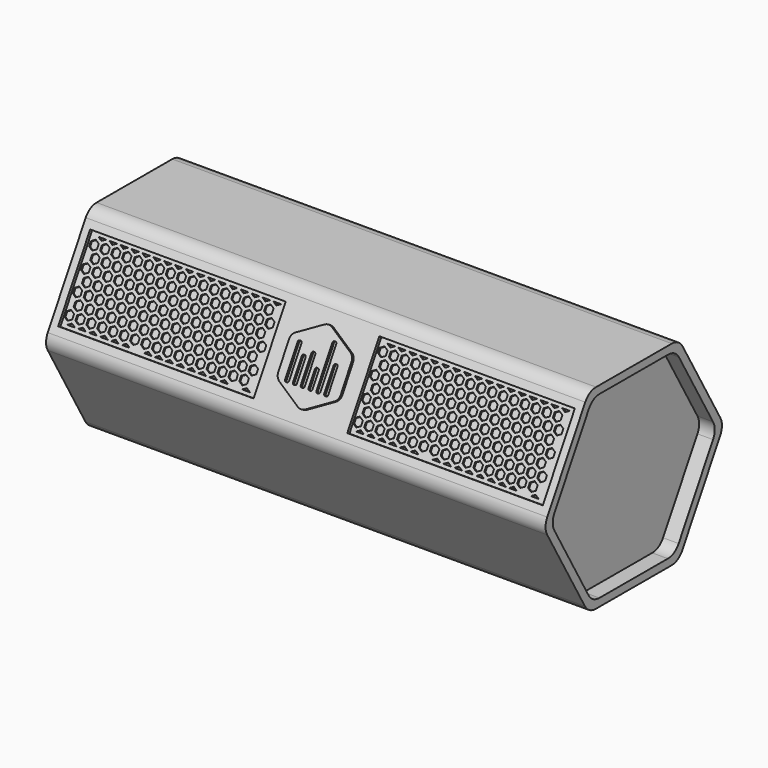
from build123d import *

# Parameters (mm, degrees)
F1_DEPTH  = 320
F3_DEPTH  = 1.5
F4_R      = 10
F6_DEPTH  = 10
F8_DEPTH  = 10
F9_R      = 10
F10_R     = 5
F11_W     = 125.25
F11_H     = 51.1217782649
F12_DEPTH = 3
F13_DEPTH = 3
F14_DEPTH = 1
F16_DEPTH = 1
F18_W     = 2.5
F18_H     = 22
F18_H_2   = 16
F18_H_3   = 19
F18_H_4   = 12
F18_H_5   = 27.5
F18_H_6   = 17
F19_DEPTH = 2
F20_R     = 1


with BuildPart() as f1:
    # F0 (on Right) → F1 (new body)
    with BuildSketch(Plane.YZ):
        Polygon((-35.9565990903, 62.5736071774), (-72.1686329672, 0.1474753428), (-36.2120338769, -62.4261318346), (35.9565990903, -62.5736071774), (72.1686329672, -0.1474753428), (36.2120338769, 62.4261318346), align=None)
    extrude(amount=F1_DEPTH)

    # F4
    f4_edges = [f1.edges().sort_by_distance(p)[0] for p in [
        (160, 36.212034, 62.426132),
        (160, -35.956599, 62.573607),
        (160, -72.168633, 0.147475),
        (160, -36.212034, -62.426132),
        (160, 35.956599, -62.573607),
        (160, 72.168633, -0.147475),
    ]]
    fillet(f4_edges, radius=F4_R)

    # F5 (on face) → F6 (cut)
    with BuildSketch(Plane(origin=(0, 0, 0), x_dir=(0, -1, 0), z_dir=(-1, 0, 0))):
        Polygon((33.207939238, 57.4942419201), (-33.1875044551, 57.5060399475), (-66.3954436931, 0.0117980274), (-33.207939238, -57.4942419201), (33.1875044551, -57.5060399475), (66.3954436931, -0.0117980274), align=None)
    extrude(amount=-F6_DEPTH, mode=Mode.SUBTRACT)

    # F7 (on face) → F8 (cut)
    with BuildSketch(Plane.YZ.offset(320)):
        Polygon((33.3252825309, 57.4261318346), (-33.0698477444, 57.5736071774), (-66.3951302753, 0.1474753428), (-33.3252825309, -57.4261318346), (33.0698477444, -57.5736071774), (66.3951302753, -0.1474753428), align=None)
    extrude(amount=-F8_DEPTH, mode=Mode.SUBTRACT)

    # F9
    f9_edges = [f1.edges().sort_by_distance(p)[0] for p in [
        (5, 33.187504, 57.50604),
        (5, 66.395444, 0.011798),
        (5, -33.207939, 57.494242),
        (5, -66.395444, -0.011798),
        (5, -33.187504, -57.50604),
        (5, 33.207939, -57.494242),
        (315, 33.325283, 57.426132),
        (315, 66.39513, -0.147475),
        (315, -33.069848, 57.573607),
        (315, -66.39513, 0.147475),
        (315, -33.325283, -57.426132),
        (315, 33.069848, -57.573607),
    ]]
    fillet(f9_edges, radius=F9_R)

    # F11 (on face) → F12 (cut)
    with BuildSketch(Plane(origin=(0, -54.0626160288, 31.3605412601), x_dir=(1, 0, 0), z_dir=(0, -0.8650018565, 0.5017686602))):
        with Locations((67.375, 0)):
            Rectangle(F11_W, F11_H)
    extrude(amount=-F12_DEPTH, mode=Mode.SUBTRACT)

    # F11 (on face) → F13 (cut)
    with BuildSketch(Plane(origin=(0, -54.0626160288, 31.3605412601), x_dir=(1, 0, 0), z_dir=(0, -0.8650018565, 0.5017686602))):
        with Locations((252.625, 0)):
            Rectangle(F11_W, F11_H)
    extrude(amount=-F13_DEPTH, mode=Mode.SUBTRACT)


with BuildPart() as f3:
    # F2 (on face) → F3 (new body)
    with BuildSketch(Plane(origin=(0, -54.0626160288, 31.3605412601), x_dir=(1, 0, 0), z_dir=(0, -0.8650018565, 0.5017686602))):
        Polygon((159.8552660133, 23.0669244835), (139.9510904167, 11.4081189325), (140.0958244034, -11.658805551), (160.1447339867, -23.0669244835), (180.0489095833, -11.4081189325), (179.9041755966, 11.658805551), align=None)
    extrude(amount=F3_DEPTH)

    # F10
    f10_edges = [f3.edges().sort_by_distance(p)[0] for p in [
        (159.855266, -43.137108, 51.6898),
        (179.904176, -48.861344, 41.821756),
        (180.04891, -60.435604, 21.868824),
        (160.144734, -66.285627, 11.783935),
        (140.095824, -60.561391, 21.651979),
        (139.95109, -48.987131, 41.604912),
    ]]
    fillet(f10_edges, radius=F10_R)

    # F18 (on face) → F19 (cut)
    with BuildSketch(Plane(origin=(0, -55.3601188135, 32.1131942503), x_dir=(1, 0, 0), z_dir=(0, -0.8650018565, 0.5017686602))):
        with Locations((146.6441166401, -1.09411787)):
            Rectangle(F18_W, F18_H)
        with Locations((151.6441166401, -4.0627452467)):
            Rectangle(F18_W, F18_H_2)
        with Locations((156.6441166401, -2.5313726233)):
            Rectangle(F18_W, F18_H_3)
        with Locations((161.6441166401, -6)):
            Rectangle(F18_W, F18_H_4)
        with Locations((166.6441166401, 1.7813726233)):
            Rectangle(F18_W, F18_H_5)
        with Locations((171.6441166401, -3.4372547533)):
            Rectangle(F18_W, F18_H_6)
    extrude(amount=-F19_DEPTH, mode=Mode.SUBTRACT)

    # F20
    f20_edges = [f3.edges().sort_by_distance(p)[0] for p in [
        (145.394117, -49.740906, 40.305474),
        (147.894117, -49.740906, 40.305474),
        (145.394117, -60.779817, 21.275433),
        (147.894117, -60.779817, 21.275433),
        (150.394117, -52.735776, 35.1426),
        (152.894117, -52.735776, 35.1426),
        (152.894117, -60.764075, 21.302571),
        (150.394117, -60.764075, 21.302571),
        (155.394117, -51.214729, 37.764743),
        (157.894117, -51.214729, 37.764743),
        (157.894117, -60.748333, 21.329708),
        (155.394117, -60.748333, 21.329708),
        (160.394117, -54.711367, 31.736868),
        (162.894117, -54.711367, 31.736868),
        (162.894117, -60.732591, 21.356845),
        (160.394117, -60.732591, 21.356845),
        (165.394117, -46.918211, 45.171534),
        (167.894117, -46.918211, 45.171534),
        (167.894117, -60.71685, 21.383983),
        (165.394117, -60.71685, 21.383983),
        (172.894117, -52.171041, 36.116152),
        (170.394117, -52.171041, 36.116152),
        (172.894117, -60.701108, 21.41112),
        (170.394117, -60.701108, 21.41112),
    ]]
    fillet(f20_edges, radius=F20_R)


with BuildPart() as f14:
    # F14 (new): a face of the model
    f14_faces = [f1.part.faces().sort_by_distance(p)[0] for p in [
        (67.375, -51.4676104594, 29.8552352796),
    ]]
    extrude(f14_faces, amount=F14_DEPTH)

    # F15 (on face) → F16 (cut)
    with BuildSketch(Plane(origin=(0, -52.3326123159, 30.3570039398), x_dir=(1, 0, 0), z_dir=(0, -0.8650018565, 0.5017686602))):
        Polygon((69.875, -1.443375673), (69.875, 1.443375673), (67.375, 2.8867513459), (64.875, 1.443375673), (64.875, -1.443375673), (67.375, -2.8867513459), align=None)
        Polygon((74.3182979262, 2.8861944162), (71.8471312784, 1.3939917717), (71.9038333522, -1.4922026445), (74.4317020738, -2.8861944162), (76.9028687216, -1.3939917717), (76.8461666478, 1.4922026445), align=None)
        Polygon((81.375, 2.8867513459), (78.875, 1.443375673), (78.875, -1.443375673), (81.375, -2.8867513459), (83.875, -1.443375673), (83.875, 1.443375673), align=None)
        Polygon((88.375, 2.886751346), (85.875, 1.443375673), (85.875, -1.443375673), (88.375, -2.8867513459), (90.875, -1.443375673), (90.875, 1.443375673), align=None)
        Polygon((95.375, 2.8867513459), (92.875, 1.443375673), (92.875, -1.443375673), (95.375, -2.8867513459), (97.875, -1.443375673), (97.875, 1.443375673), align=None)
        Polygon((102.375, 2.8867513459), (99.875, 1.443375673), (99.875, -1.443375673), (102.375, -2.886751346), (104.875, -1.443375673), (104.875, 1.443375673), align=None)
        Polygon((109.375, 2.8867513459), (106.875, 1.443375673), (106.875, -1.443375673), (109.375, -2.8867513459), (111.875, -1.443375673), (111.875, 1.443375673), align=None)
        Polygon((116.375, 2.8867513459), (113.875, 1.443375673), (113.875, -1.443375673), (116.375, -2.8867513459), (118.875, -1.443375673), (118.875, 1.443375673), align=None)
        Polygon((123.375, 2.8867513459), (120.875, 1.4433756729), (120.875, -1.443375673), (123.375, -2.886751346), (125.875, -1.443375673), (125.875, 1.4433756729), align=None)
        Polygon((22.875, -1.443375673), (25.375, -2.8867513459), (27.875, -1.443375673), (27.875, 1.443375673), (25.375, 2.8867513459), (22.875, 1.443375673), align=None)
        Polygon((20.875, -1.443375673), (20.875, 1.443375673), (18.375, 2.8867513459), (15.875, 1.443375673), (15.875, -1.443375673), (18.375, -2.8867513459), align=None)
        Polygon((29.875, -1.443375673), (32.375, -2.886751346), (34.875, -1.443375673), (34.875, 1.443375673), (32.375, 2.8867513459), (29.875, 1.443375673), align=None)
        Polygon((13.875, 1.4433756729), (11.375, 2.8867513459), (8.875, 1.4433756729), (8.875, -1.443375673), (11.375, -2.886751346), (13.875, -1.443375673), align=None)
        Polygon((48.875, 1.443375673), (46.375, 2.886751346), (43.875, 1.443375673), (43.875, -1.443375673), (46.375, -2.8867513459), (48.875, -1.443375673), align=None)
        Polygon((50.875, -1.443375673), (53.375, -2.8867513459), (55.875, -1.443375673), (55.875, 1.443375673), (53.375, 2.8867513459), (50.875, 1.443375673), align=None)
        Polygon((41.875, -1.443375673), (41.875, 1.443375673), (39.375, 2.8867513459), (36.875, 1.443375673), (36.875, -1.443375673), (39.375, -2.8867513459), align=None)
        Polygon((62.9028687216, 1.3939917717), (60.4317020738, 2.8861944162), (57.9038333522, 1.4922026445), (57.8471312784, -1.3939917717), (60.3182979262, -2.8861944162), (62.8461666478, -1.4922026445), align=None)
        Polygon((50.2418052453, 9.1463911622), (47.7418052453, 7.7030154892), (47.7418052453, 4.8162641432), (50.2418052453, 3.3728884703), (52.7418052453, 4.8162641432), (52.7418052453, 7.7030154892), align=None)
        Polygon((106.2418052453, 9.1463911622), (103.7418052453, 7.7030154892), (103.7418052453, 4.8162641432), (106.2418052453, 3.3728884703), (108.7418052453, 4.8162641432), (108.7418052453, 7.7030154892), align=None)
        Polygon((8.2418052453, 9.1463911621), (8.2418052453, 3.3728884702), (10.7418052453, 4.8162641432), (10.7418052453, 7.7030154892), align=None)
        Polygon((5.7418052453, 4.8162641432), (8.2418052453, 3.3728884702), (8.2418052453, 9.1463911621), (5.7418052453, 7.7030154891), align=None)
        Polygon((117.7418052453, 4.8162641432), (120.2418052452, 3.3728884702), (122.7418052452, 4.8162641432), (122.7418052453, 7.7030154891), (120.2418052453, 9.1463911621), (117.7418052453, 7.7030154892), align=None)
        Polygon((22.2418052453, 9.1463911622), (19.7418052453, 7.7030154892), (19.7418052453, 4.8162641432), (22.2418052453, 3.3728884703), (24.7418052453, 4.8162641432), (24.7418052453, 7.7030154892), align=None)
        Polygon((38.7418052453, 4.8162641433), (38.7418052453, 7.7030154892), (36.2418052453, 9.1463911622), (33.7418052453, 7.7030154892), (33.7418052453, 4.8162641432), (36.2418052453, 3.3728884703), align=None)
        Polygon((92.2418052453, 9.1463911622), (89.7418052453, 7.7030154892), (89.7418052453, 4.8162641433), (92.2418052453, 3.3728884703), (94.7418052453, 4.8162641432), (94.7418052453, 7.7030154892), align=None)
        Polygon((99.2418052453, 9.1463911622), (96.7418052453, 7.7030154892), (96.7418052453, 4.8162641432), (99.2418052453, 3.3728884703), (101.7418052453, 4.8162641432), (101.7418052453, 7.7030154892), align=None)
        Polygon((64.2418052453, 3.3728884703), (66.7418052453, 4.8162641433), (66.7418052453, 7.7030154892), (64.2418052453, 9.1463911622), (61.7418052453, 7.7030154892), (61.7418052453, 4.8162641432), align=None)
        Polygon((115.7418052453, 4.8162641432), (115.7418052453, 7.7030154892), (113.2418052453, 9.1463911622), (110.7418052453, 7.7030154892), (110.7418052453, 4.8162641432), (113.2418052453, 3.3728884703), align=None)
        Polygon((43.2418052453, 9.1463911622), (40.7418052453, 7.7030154892), (40.7418052453, 4.8162641433), (43.2418052453, 3.3728884703), (45.7418052453, 4.8162641433), (45.7418052453, 7.7030154892), align=None)
        Polygon((82.7418052453, 4.8162641433), (85.2418052453, 3.3728884703), (87.7418052453, 4.8162641433), (87.7418052453, 7.7030154892), (85.2418052453, 9.1463911622), (82.7418052453, 7.7030154892), align=None)
        Polygon((75.7418052453, 4.8162641432), (78.2418052453, 3.3728884703), (80.7418052453, 4.8162641432), (80.7418052453, 7.7030154892), (78.2418052453, 9.1463911622), (75.7418052453, 7.7030154892), align=None)
        Polygon((59.712971893, 4.7674371717), (59.7696739669, 7.6536315879), (57.2985073191, 9.1458342324), (54.7706385975, 7.7518424607), (54.7139365236, 4.8656480445), (57.1851031714, 3.3734454), align=None)
        Polygon((26.7418052453, 4.8162641432), (29.2418052453, 3.3728884703), (31.7418052453, 4.8162641432), (31.7418052453, 7.7030154892), (29.2418052453, 9.1463911622), (26.7418052453, 7.7030154892), align=None)
        Polygon((17.7418052453, 7.7030154892), (15.2418052453, 9.1463911622), (12.7418052453, 7.7030154892), (12.7418052453, 4.8162641432), (15.2418052453, 3.3728884703), (17.7418052453, 4.8162641432), align=None)
        Polygon((71.2985073191, 3.3734454), (73.7696739669, 4.8656480445), (73.712971893, 7.7518424607), (71.1851031714, 9.1458342324), (68.7139365236, 7.6536315879), (68.7706385975, 4.7674371717), align=None)
        Polygon((123.7049438918, 9.5428702504), (126.2049438918, 10.9862459233), (126.2049438918, 13.8729972693), (123.7049438918, 15.3163729422), (121.2049438918, 13.8729972693), (121.2049438918, 10.9862459233), align=None)
        Polygon((32.7049438918, 15.3163729423), (30.2049438918, 13.8729972693), (30.2049438918, 10.9862459234), (32.7049438918, 9.5428702504), (35.2049438918, 10.9862459234), (35.2049438918, 13.8729972693), align=None)
        Polygon((116.7049438918, 9.5428702504), (119.2049438918, 10.9862459234), (119.2049438918, 13.8729972693), (116.7049438918, 15.3163729423), (114.2049438918, 13.8729972693), (114.2049438918, 10.9862459234), align=None)
        Polygon((27.0717491371, 17.2458857396), (29.5717491371, 15.8025100666), (32.0717491371, 17.2458857396), (32.0717491371, 20.1326370855), (29.5717491371, 21.5760127585), (27.0717491371, 20.1326370855), align=None)
        Polygon((56.2049438918, 10.9862459234), (56.2049438918, 13.8729972693), (53.7049438918, 15.3163729423), (51.2049438918, 13.8729972693), (51.2049438918, 10.9862459234), (53.7049438918, 9.5428702504), align=None)
        Polygon((18.7049438918, 9.5428702504), (21.2049438918, 10.9862459234), (21.2049438918, 13.8729972693), (18.7049438918, 15.3163729423), (16.2049438918, 13.8729972693), (16.2049438918, 10.9862459234), align=None)
        Polygon((88.7049438918, 9.5428702504), (91.2049438918, 10.9862459234), (91.2049438918, 13.8729972693), (88.7049438918, 15.3163729423), (86.2049438918, 13.8729972693), (86.2049438918, 10.9862459234), align=None)
        Polygon((22.5717491371, 21.5760127585), (20.0717491371, 20.1326370855), (20.0717491371, 17.2458857396), (22.5717491371, 15.8025100666), (25.0717491371, 17.2458857396), (25.0717491371, 20.1326370855), align=None)
        Polygon((120.5717491371, 15.8025100666), (123.0717491371, 17.2458857395), (123.0717491371, 20.1326370855), (120.5717491371, 21.5760127585), (118.0717491371, 20.1326370855), (118.0717491371, 17.2458857396), align=None)
        Polygon((23.2049438918, 10.9862459234), (25.7049438918, 9.5428702504), (28.2049438918, 10.9862459234), (28.2049438918, 13.8729972693), (25.7049438918, 15.3163729423), (23.2049438918, 13.8729972693), align=None)
        Polygon((37.2049438918, 13.8729972693), (37.2049438918, 10.9862459234), (39.7049438918, 9.5428702504), (42.2049438918, 10.9862459234), (42.2049438918, 13.8729972693), (39.7049438918, 15.3163729423), align=None)
        Polygon((49.2049438918, 10.9862459234), (49.2049438918, 13.8729972693), (46.7049438918, 15.3163729423), (44.2049438918, 13.8729972693), (44.2049438918, 10.9862459234), (46.7049438918, 9.5428702504), align=None)
        Polygon((11.7049438918, 15.3163729422), (9.2049438918, 13.8729972693), (9.2049438919, 10.9862459233), (11.7049438919, 9.5428702504), (14.2049438918, 10.9862459233), (14.2049438918, 13.8729972693), align=None)
        Polygon((83.0717491371, 17.2458857396), (85.5717491371, 15.8025100666), (88.0717491371, 17.2458857396), (88.0717491371, 20.1326370855), (85.5717491371, 21.5760127585), (83.0717491371, 20.1326370855), align=None)
        Polygon((81.7049438918, 15.3163729423), (79.2049438918, 13.8729972693), (79.2049438918, 10.9862459234), (81.7049438918, 9.5428702504), (84.2049438918, 10.9862459234), (84.2049438918, 13.8729972693), align=None)
        Polygon((60.7616459657, 15.3158160125), (58.2337772441, 13.9218242408), (58.1770751702, 11.0356298246), (60.648241818, 9.5434271801), (63.1761105396, 10.9374189518), (63.2328126135, 13.8236133681), align=None)
        Polygon((74.0429157849, 20.1814640571), (71.5150470633, 21.5754558288), (69.0438804155, 20.0832531843), (69.1005824893, 17.1970587681), (71.6284512109, 15.8030669964), (74.0996178587, 17.2952696408), align=None)
        Polygon((50.5717491371, 15.8025100666), (53.0717491371, 17.2458857396), (53.0717491371, 20.1326370855), (50.5717491371, 21.5760127585), (48.0717491371, 20.1326370855), (48.0717491371, 17.2458857396), align=None)
        Polygon((65.2049438918, 10.9862459234), (67.7049438918, 9.5428702504), (70.2049438918, 10.9862459234), (70.2049438918, 13.8729972693), (67.7049438918, 15.3163729423), (65.2049438918, 13.8729972693), align=None)
        Polygon((109.0717491371, 17.2458857396), (109.0717491371, 20.1326370855), (106.5717491371, 21.5760127585), (104.0717491371, 20.1326370855), (104.0717491371, 17.2458857396), (106.5717491371, 15.8025100666), align=None)
        Polygon((102.7049438918, 9.5428702504), (105.2049438918, 10.9862459234), (105.2049438918, 13.8729972693), (102.7049438918, 15.3163729423), (100.2049438918, 13.8729972693), (100.2049438918, 10.9862459234), align=None)
        Polygon((43.5717491371, 21.5760127585), (41.0717491371, 20.1326370855), (41.0717491371, 17.2458857396), (43.5717491371, 15.8025100666), (46.0717491371, 17.2458857396), (46.0717491371, 20.1326370855), align=None)
        Polygon((112.2049438918, 13.8729972693), (109.7049438918, 15.3163729423), (107.2049438918, 13.8729972693), (107.2049438918, 10.9862459234), (109.7049438918, 9.5428702504), (112.2049438918, 10.9862459234), align=None)
        Polygon((67.0717491371, 20.1326370855), (64.5717491371, 21.5760127585), (62.0717491371, 20.1326370855), (62.0717491371, 17.2458857396), (64.5717491371, 15.8025100666), (67.0717491371, 17.2458857396), align=None)
        Polygon((18.0717491371, 20.1326370855), (15.5717491371, 21.5760127585), (13.0717491371, 20.1326370855), (13.0717491371, 17.2458857396), (15.5717491371, 15.8025100666), (18.0717491371, 17.2458857396), align=None)
        Polygon((98.2049438918, 13.8729972693), (95.7049438918, 15.3163729423), (93.2049438918, 13.8729972693), (93.2049438918, 10.9862459234), (95.7049438918, 9.5428702504), (98.2049438918, 10.9862459234), align=None)
        Polygon((92.5717491371, 15.8025100666), (95.0717491371, 17.2458857396), (95.0717491371, 20.1326370855), (92.5717491371, 21.5760127585), (90.0717491371, 20.1326370855), (90.0717491371, 17.2458857396), align=None)
        Polygon((72.2337772441, 10.9374189519), (74.7616459657, 9.5434271801), (77.2328126135, 11.0356298246), (77.1761105396, 13.9218242408), (74.648241818, 15.3158160125), (72.1770751702, 13.8236133681), align=None)
        Polygon((55.0438804155, 17.2952696408), (57.5150470633, 15.8030669964), (60.0429157849, 17.1970587681), (60.0996178587, 20.0832531843), (57.6284512109, 21.5754558288), (55.1005824893, 20.1814640571), align=None)
        Polygon((81.0717491371, 20.1326370855), (78.5717491371, 21.5760127585), (76.0717491371, 20.1326370855), (76.0717491371, 17.2458857396), (78.5717491371, 15.8025100666), (81.0717491371, 17.2458857396), align=None)
        Polygon((8.5717491371, 21.5760127585), (6.0717491371, 20.1326370855), (6.0717491371, 17.2458857395), (8.5717491371, 15.8025100666), align=None)
        Polygon((11.0717491371, 20.1326370855), (8.5717491371, 21.5760127585), (8.5717491371, 15.8025100666), (11.0717491371, 17.2458857396), align=None)
        Polygon((99.5717491371, 21.5760127585), (97.0717491371, 20.1326370855), (97.0717491371, 17.2458857396), (99.5717491371, 15.8025100666), (102.0717491371, 17.2458857396), (102.0717491371, 20.1326370855), align=None)
        Polygon((36.5717491371, 15.8025100666), (39.0717491371, 17.2458857396), (39.0717491371, 20.1326370855), (36.5717491371, 21.5760127585), (34.0717491371, 20.1326370855), (34.0717491371, 17.2458857396), align=None)
        Polygon((111.0717491371, 17.2458857396), (113.5717491371, 15.8025100666), (116.0717491371, 17.2458857396), (116.0717491371, 20.1326370855), (113.5717491371, 21.5760127585), (111.0717491371, 20.1326370855), align=None)
        Polygon((124.0348877837, 21.9724918467), (126.5348877837, 23.4158675197), (121.5348877837, 23.4158675197), align=None)
        Polygon((117.0348877837, 21.9724918467), (119.5348877837, 23.4158675197), (114.5348877837, 23.4158675197), align=None)
        Polygon((56.5348877837, 23.4158675197), (51.5348877837, 23.4158675197), (54.0348877837, 21.9724918467), align=None)
        Polygon((89.0348877837, 21.9724918467), (91.5348877837, 23.4158675197), (86.5348877837, 23.4158675197), align=None)
        Polygon((23.5348877837, 23.4158675197), (26.0348877837, 21.9724918467), (28.5348877837, 23.4158675197), align=None)
        Polygon((42.5348877837, 23.4158675197), (37.5348877837, 23.4158675197), (40.0348877837, 21.9724918467), align=None)
        Polygon((49.5348877837, 23.4158675197), (44.5348877837, 23.4158675197), (47.0348877837, 21.9724918467), align=None)
        Polygon((21.5348877837, 23.4158675197), (16.5348877837, 23.4158675197), (19.0348877837, 21.9724918467), align=None)
        Polygon((79.5348877837, 23.4158675197), (82.0348877837, 21.9724918467), (84.5348877837, 23.4158675197), align=None)
        Polygon((65.5348877837, 23.4158675197), (68.0348877837, 21.9724918467), (70.5348877837, 23.4158675197), align=None)
        Polygon((103.0348877837, 21.9724918467), (105.5348877837, 23.4158675197), (100.5348877837, 23.4158675197), align=None)
        Polygon((63.5060544315, 23.3670405482), (58.5070190621, 23.465251421), (60.9781857099, 21.9730487765), align=None)
        Polygon((110.0348877837, 21.9724918467), (112.5348877837, 23.4158675197), (107.5348877837, 23.4158675197), align=None)
        Polygon((93.5348877837, 23.4158675197), (96.0348877837, 21.9724918467), (98.5348877837, 23.4158675197), align=None)
        Polygon((72.5637211359, 23.3670405482), (75.0915898575, 21.9730487765), (77.5627565053, 23.465251421), align=None)
        Polygon((9.5348877837, 23.4158675197), (12.0348877837, 21.9724918467), (14.5348877837, 23.4158675197), align=None)
        Polygon((30.5348877837, 23.4158675197), (33.0348877837, 21.9724918467), (35.5348877837, 23.4158675197), align=None)
        Polygon((24.4695560985, -7.6147549784), (24.4695560985, -4.7280036324), (21.9695560985, -3.2846279594), (19.4695560985, -4.7280036324), (19.4695560985, -7.6147549784), (21.9695560985, -9.0581306513), align=None)
        Polygon((77.9695560985, -3.2846279594), (75.4695560985, -4.7280036324), (75.4695560985, -7.6147549784), (77.9695560985, -9.0581306513), (80.4695560985, -7.6147549784), (80.4695560985, -4.7280036324), align=None)
        Polygon((54.4983894507, -4.6791766609), (54.4416873769, -7.5653710771), (56.9128540247, -9.0575737216), (59.4407227463, -7.6635819499), (59.4974248201, -4.7773875337), (57.0262581724, -3.2851848892), align=None)
        Polygon((46.1027508533, -15.3177704676), (48.6027508533, -13.8743947946), (48.6027508533, -10.9876434486), (46.1027508533, -9.5442677757), (43.6027508533, -10.9876434486), (43.6027508533, -13.8743947946), align=None)
        Polygon((20.6027508533, -13.8743947946), (20.6027508533, -10.9876434486), (18.1027508533, -9.5442677757), (15.6027508533, -10.9876434486), (15.6027508533, -13.8743947946), (18.1027508533, -15.3177704676), align=None)
        Polygon((50.6027508533, -13.8743947946), (53.1027508533, -15.3177704676), (55.6027508533, -13.8743947946), (55.6027508533, -10.9876434486), (53.1027508533, -9.5442677757), (50.6027508533, -10.9876434486), align=None)
        Polygon((110.4695560985, -4.7280036324), (110.4695560985, -7.6147549784), (112.9695560985, -9.0581306513), (115.4695560985, -7.6147549784), (115.4695560985, -4.7280036324), (112.9695560985, -3.2846279594), align=None)
        Polygon((61.4695560985, -4.7280036324), (61.4695560985, -7.6147549784), (63.9695560985, -9.0581306513), (66.4695560985, -7.6147549784), (66.4695560985, -4.7280036324), (63.9695560985, -3.2846279594), align=None)
        Polygon((94.4695560985, -7.6147549784), (94.4695560985, -4.7280036324), (91.9695560985, -3.2846279594), (89.4695560985, -4.7280036324), (89.4695560985, -7.6147549784), (91.9695560985, -9.0581306513), align=None)
        Polygon((7.9695560985, -3.2846279595), (5.4695560985, -4.7280036325), (5.4695560985, -7.6147549784), (7.9695560985, -9.0581306514), align=None)
        Polygon((10.4695560985, -4.7280036325), (7.9695560985, -3.2846279595), (7.9695560985, -9.0581306514), (10.4695560985, -7.6147549784), align=None)
        Polygon((40.4695560985, -4.7280036324), (40.4695560985, -7.6147549784), (42.9695560985, -9.0581306513), (45.4695560985, -7.6147549784), (45.4695560985, -4.7280036324), (42.9695560985, -3.2846279594), align=None)
        Polygon((105.9695560985, -3.2846279595), (103.4695560985, -4.7280036324), (103.4695560985, -7.6147549784), (105.9695560985, -9.0581306513), (108.4695560985, -7.6147549784), (108.4695560985, -4.7280036324), align=None)
        Polygon((74.1594529271, -15.3172135378), (76.6306195749, -13.8250108933), (76.573917501, -10.9388164771), (74.0460487794, -9.5448247054), (71.5748821316, -11.0370273499), (71.6315842055, -13.9232217661), align=None)
        Polygon((99.6027508533, -13.8743947946), (102.1027508533, -15.3177704676), (104.6027508533, -13.8743947946), (104.6027508533, -10.9876434486), (102.1027508533, -9.5442677757), (99.6027508533, -10.9876434487), align=None)
        Polygon((73.4974248201, -7.5653710771), (73.4407227463, -4.6791766609), (70.9128540247, -3.2851848892), (68.4416873769, -4.7773875337), (68.4983894507, -7.6635819499), (71.0262581724, -9.0575737216), align=None)
        Polygon((39.1027508533, -9.5442677757), (36.6027508533, -10.9876434486), (36.6027508533, -13.8743947946), (39.1027508533, -15.3177704676), (41.6027508533, -13.8743947946), (41.6027508533, -10.9876434486), align=None)
        Polygon((67.1027508533, -9.5442677757), (64.6027508533, -10.9876434486), (64.6027508533, -13.8743947946), (67.1027508533, -15.3177704676), (69.6027508533, -13.8743947946), (69.6027508533, -10.9876434486), align=None)
        Polygon((32.1027508533, -15.3177704676), (34.6027508533, -13.8743947946), (34.6027508533, -10.9876434487), (32.1027508533, -9.5442677757), (29.6027508533, -10.9876434486), (29.6027508533, -13.8743947946), align=None)
        Polygon((57.5748821317, -13.8250108933), (60.0460487794, -15.3172135378), (62.573917501, -13.9232217661), (62.6306195749, -11.0370273499), (60.1594529271, -9.5448247054), (57.6315842055, -10.9388164771), align=None)
        Polygon((13.6027508533, -10.9876434487), (11.1027508533, -9.5442677757), (8.6027508533, -10.9876434487), (8.6027508533, -13.8743947946), (11.1027508533, -15.3177704676), (13.6027508533, -13.8743947946), align=None)
        Polygon((52.4695560985, -4.7280036324), (49.9695560985, -3.2846279594), (47.4695560985, -4.7280036324), (47.4695560985, -7.6147549784), (49.9695560985, -9.0581306513), (52.4695560985, -7.6147549784), align=None)
        Polygon((122.4695560985, -4.7280036325), (119.9695560985, -3.2846279595), (117.4695560985, -4.7280036325), (117.4695560985, -7.6147549784), (119.9695560985, -9.0581306514), (122.4695560985, -7.6147549784), align=None)
        Polygon((27.6027508533, -13.8743947946), (27.6027508533, -10.9876434486), (25.1027508533, -9.5442677757), (22.6027508533, -10.9876434486), (22.6027508533, -13.8743947946), (25.1027508533, -15.3177704676), align=None)
        Polygon((28.9695560985, -3.2846279595), (26.4695560985, -4.7280036324), (26.4695560985, -7.6147549784), (28.9695560985, -9.0581306513), (31.4695560985, -7.6147549784), (31.4695560985, -4.7280036324), align=None)
        Polygon((35.9695560985, -9.0581306513), (38.4695560985, -7.6147549784), (38.4695560985, -4.7280036324), (35.9695560985, -3.2846279594), (33.4695560985, -4.7280036324), (33.4695560985, -7.6147549784), align=None)
        Polygon((118.6027508533, -10.9876434486), (116.1027508533, -9.5442677757), (113.6027508533, -10.9876434486), (113.6027508533, -13.8743947946), (116.1027508533, -15.3177704676), (118.6027508533, -13.8743947946), align=None)
        Polygon((125.6027508533, -13.8743947946), (125.6027508533, -10.9876434487), (123.1027508533, -9.5442677757), (120.6027508533, -10.9876434487), (120.6027508533, -13.8743947946), (123.1027508533, -15.3177704676), align=None)
        Polygon((109.1027508533, -15.3177704676), (111.6027508533, -13.8743947946), (111.6027508533, -10.9876434486), (109.1027508533, -9.5442677757), (106.6027508533, -10.9876434486), (106.6027508533, -13.8743947946), align=None)
        Polygon((14.9695560985, -9.0581306513), (17.4695560985, -7.6147549784), (17.4695560985, -4.7280036324), (14.9695560985, -3.2846279594), (12.4695560985, -4.7280036324), (12.4695560985, -7.6147549784), align=None)
        Polygon((95.1027508533, -15.3177704676), (97.6027508533, -13.8743947946), (97.6027508533, -10.9876434486), (95.1027508533, -9.5442677757), (92.6027508533, -10.9876434486), (92.6027508533, -13.8743947946), align=None)
        Polygon((101.4695560985, -7.6147549784), (101.4695560985, -4.7280036324), (98.9695560985, -3.2846279595), (96.4695560985, -4.7280036324), (96.4695560985, -7.6147549784), (98.9695560985, -9.0581306513), align=None)
        Polygon((82.4695560985, -7.6147549784), (84.9695560985, -9.0581306513), (87.4695560985, -7.6147549784), (87.4695560985, -4.7280036324), (84.9695560985, -3.2846279594), (82.4695560985, -4.7280036324), align=None)
        Polygon((90.6027508533, -13.8743947946), (90.6027508533, -10.9876434486), (88.1027508533, -9.5442677757), (85.6027508533, -10.9876434486), (85.6027508533, -13.8743947946), (88.1027508533, -15.3177704676), align=None)
        Polygon((81.1027508533, -9.5442677757), (78.6027508533, -10.9876434486), (78.6027508533, -13.8743947946), (81.1027508533, -15.3177704676), (83.6027508533, -13.8743947946), (83.6027508533, -10.9876434486), align=None)
        Polygon((24.1973069518, -20.0457741), (24.1973069518, -17.159022754), (21.6973069518, -15.7156470811), (19.1973069518, -17.159022754), (19.1973069518, -20.0457741), (21.6973069518, -21.489149773), align=None)
        Polygon((77.6973069518, -15.7156470811), (75.1973069518, -17.159022754), (75.1973069518, -20.0457741), (77.6973069518, -21.489149773), (80.1973069518, -20.0457741), (80.1973069518, -17.159022754), align=None)
        Polygon((54.226140304, -17.1101957825), (54.1694382302, -19.9963901987), (56.640604878, -21.4885928432), (59.1684735996, -20.0946010715), (59.2251756734, -17.2084066553), (56.7540090256, -15.7162040108), align=None)
        Polygon((15.3305017065, -23.4186625703), (20.3305017065, -23.4186625703), (17.8305017065, -21.9752868973), align=None)
        Polygon((110.1973069518, -17.159022754), (110.1973069518, -20.0457741), (112.6973069518, -21.489149773), (115.1973069518, -20.0457741), (115.1973069518, -17.159022754), (112.6973069518, -15.7156470811), align=None)
        Polygon((61.1973069518, -17.159022754), (61.1973069518, -20.0457741), (63.6973069518, -21.489149773), (66.1973069518, -20.0457741), (66.1973069518, -17.159022754), (63.6973069518, -15.7156470811), align=None)
        Polygon((94.1973069518, -20.0457741), (94.1973069518, -17.159022754), (91.6973069518, -15.7156470811), (89.1973069518, -17.159022754), (89.1973069518, -20.0457741), (91.6973069518, -21.489149773), align=None)
        Polygon((7.6973069518, -15.7156470811), (5.1973069518, -17.1590227541), (5.1973069518, -20.0457741), (7.6973069518, -21.489149773), (10.1973069518, -20.0457741), (10.1973069518, -17.1590227541), align=None)
        Polygon((40.1973069518, -17.159022754), (40.1973069518, -20.0457741), (42.6973069518, -21.489149773), (45.1973069518, -20.0457741), (45.1973069518, -17.159022754), (42.6973069518, -15.7156470811), align=None)
        Polygon((105.6973069518, -15.7156470811), (103.1973069518, -17.159022754), (103.1973069518, -20.0457741), (105.6973069518, -21.489149773), (108.1973069518, -20.0457741), (108.1973069518, -17.159022754), align=None)
        Polygon((73.2251756734, -19.9963901987), (73.1684735996, -17.1101957825), (70.640604878, -15.7162040108), (68.1694382302, -17.2084066553), (68.226140304, -20.0946010715), (70.7540090256, -21.4885928432), align=None)
        Polygon((66.8305017065, -21.9752868973), (64.3305017065, -23.4186625703), (69.3305017065, -23.4186625703), align=None)
        Polygon((13.3305017065, -23.4186625703), (10.8305017065, -21.9752868973), (8.3305017065, -23.4186625703), align=None)
        Polygon((52.1973069518, -17.159022754), (49.6973069518, -15.7156470811), (47.1973069518, -17.159022754), (47.1973069518, -20.0457741), (49.6973069518, -21.489149773), (52.1973069518, -20.0457741), align=None)
        Polygon((122.1973069518, -17.1590227541), (119.6973069518, -15.7156470811), (117.1973069518, -17.1590227541), (117.1973069518, -20.0457741), (119.6973069518, -21.489149773), (122.1973069518, -20.0457741), align=None)
        Polygon((22.3305017065, -23.4186625703), (27.3305017065, -23.4186625703), (24.8305017065, -21.9752868973), align=None)
        Polygon((28.6973069518, -15.7156470811), (26.1973069518, -17.159022754), (26.1973069518, -20.0457741), (28.6973069518, -21.489149773), (31.1973069518, -20.0457741), (31.1973069518, -17.159022754), align=None)
        Polygon((35.6973069518, -21.489149773), (38.1973069518, -20.0457741), (38.1973069518, -17.159022754), (35.6973069518, -15.7156470811), (33.1973069518, -17.159022754), (33.1973069518, -20.0457741), align=None)
        Polygon((36.3305017065, -23.4186625703), (41.3305017065, -23.4186625703), (38.8305017065, -21.9752868973), align=None)
        Polygon((48.3305017065, -23.4186625703), (45.8305017065, -21.9752868973), (43.3305017065, -23.4186625703), align=None)
        Polygon((14.6973069518, -21.489149773), (17.1973069518, -20.0457741), (17.1973069518, -17.159022754), (14.6973069518, -15.7156470811), (12.1973069518, -17.159022754), (12.1973069518, -20.0457741), align=None)
        Polygon((101.1973069518, -20.0457741), (101.1973069518, -17.159022754), (98.6973069518, -15.7156470811), (96.1973069518, -17.159022754), (96.1973069518, -20.0457741), (98.6973069518, -21.489149773), align=None)
        Polygon((82.1973069518, -20.0457741), (84.6973069518, -21.489149773), (87.1973069518, -20.0457741), (87.1973069518, -17.159022754), (84.6973069518, -15.7156470811), (82.1973069518, -17.159022754), align=None)
        Polygon((76.3016683543, -23.3698355988), (73.7737996327, -21.975843827), (71.3026329849, -23.4680464715), align=None)
        Polygon((104.3305017065, -23.4186625703), (101.8305017065, -21.9752868973), (99.3305017065, -23.4186625703), align=None)
        Polygon((80.8305017065, -21.9752868973), (78.3305017065, -23.4186625703), (83.3305017065, -23.4186625703), align=None)
        Polygon((108.8305017065, -21.9752868973), (106.3305017065, -23.4186625703), (111.3305017065, -23.4186625703), align=None)
        Polygon((57.3593350587, -23.3698355988), (62.3583704281, -23.4680464715), (59.8872037804, -21.975843827), align=None)
        Polygon((29.3305017065, -23.4186625703), (34.3305017065, -23.4186625703), (31.8305017065, -21.9752868973), align=None)
        Polygon((90.3305017065, -23.4186625703), (87.8305017065, -21.9752868973), (85.3305017065, -23.4186625703), align=None)
        Polygon((97.3305017065, -23.4186625703), (94.8305017065, -21.9752868973), (92.3305017065, -23.4186625703), align=None)
        Polygon((122.8305017065, -21.9752868973), (120.3305017065, -23.4186625703), (125.3305017065, -23.4186625703), align=None)
    extrude(amount=-F16_DEPTH, mode=Mode.SUBTRACT)


with BuildPart() as f17_1:
    # F17: copy of F14
    add(f14.part.moved(Location((185, 0, 0))))


solid = Compound([f1.part, f3.part, f14.part, f17_1.part])
